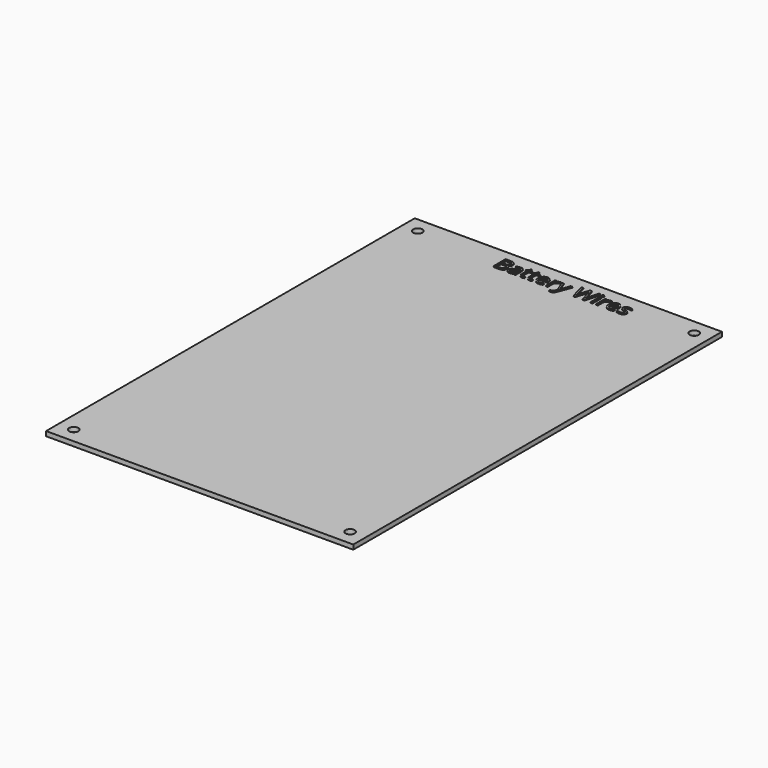
from build123d import *

# Parameters (mm, degrees)
F0_W         = 101.6
F0_H         = 152.4
F0_R         = 1.524
F1_DEPTH     = 1.524
F2_TEXT_SIZE = 7.0555555556
F3_DEPTH     = 0.254


# Not quite as in the source:
# - Text() gives the source's letters only with a copy of the font that has no kerning and outlines rounded to 1/6400 em; it was checked with that copy


with BuildPart() as f1:
    # F0 (on Top) → F1 (new body)
    with BuildSketch(Plane.XY):
        Rectangle(F0_W, F0_H)
        with Locations((-45.72, -71.12)):
            Circle(F0_R, mode=Mode.SUBTRACT)
        with Locations((45.72, -71.12)):
            Circle(F0_R, mode=Mode.SUBTRACT)
        with Locations((-45.72, 71.12)):
            Circle(F0_R, mode=Mode.SUBTRACT)
        with Locations((45.72, 71.12)):
            Circle(F0_R, mode=Mode.SUBTRACT)
    extrude(amount=F1_DEPTH)

    # F2 (on face) → F3 (join)
    with BuildSketch(Plane.XY.offset(1.524)):
        with Locations((-18.5741699347, 67.5943091172)):
            Text('Battery Wires', F2_TEXT_SIZE, font='Open Sans', text_align=(TextAlign.LEFT, TextAlign.BOTTOM))
    extrude(amount=F3_DEPTH)


solid = f1.part
